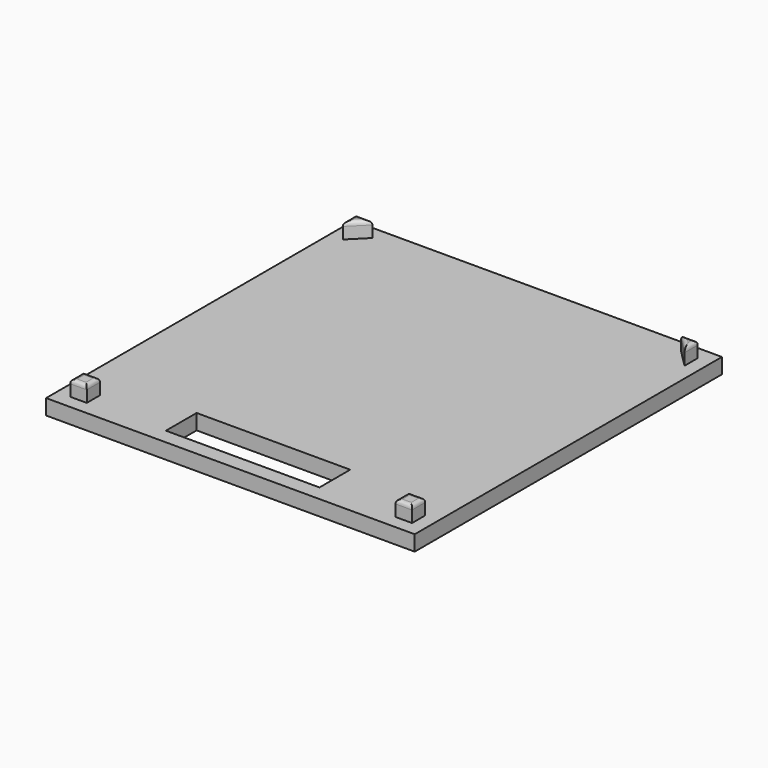
from build123d import *

# Parameters (mm, degrees)
F0_W         = 48
F0_H         = 50
F1_DEPTH     = 2
F3_DEPTH     = 2
F4_W         = 20
F4_H         = 5
F5_DEPTH     = 25
F6_T1_DEPTH  = 4.6464466094
F6_T3_DEPTH  = 4.6464466094
F6_T5_DEPTH  = 4.6464466094
F6_T7_DEPTH  = 5.5355339059
F6_T9_DEPTH  = 5.5355339059
F6_T11_DEPTH = 4.6464466094


# Not quite as in the source:
# - a fillet or chamfer that OpenCascade refuses, or shapes differently, is made with other operations: its cross-section is extruded or revolved along the edge and cut away or added
# - a feature names something its author has since deleted; it is built from what else it names


with BuildPart() as f1:
    # F0 (on Top) → F1 (new body)
    with BuildSketch(Plane.XY):
        with Locations((24, -25)):
            Rectangle(F0_W, F0_H)
    extrude(amount=F1_DEPTH)

    # F2 (on face) → F3 (join)
    with BuildSketch(Plane.XY.offset(2)):
        Polygon((1.75, -1.75), (1.75, -3.8964466094), (3.8964466094, -1.75), align=None)
        Polygon((44.1035533906, -1.75), (46.25, -3.8964466094), (46.25, -1.75), align=None)
        Polygon((46.25, -48.25), (46.25, -46.1035533906), (44.1035533906, -48.25), align=None)
        Polygon((3.8964466094, -48.25), (1.75, -46.1035533906), (1.75, -48.25), align=None)
        Polygon((3.8964466094, -46.1035533906), (1.75, -46.1035533906), (3.8964466094, -48.25), align=None)
        Polygon((44.1035533906, -48.25), (46.25, -46.1035533906), (44.1035533906, -46.1035533906), align=None)
    extrude(amount=F3_DEPTH)

    # F4 (on face) → F5 (cut)
    with BuildSketch(Plane.XY.offset(2)):
        with Locations((24, -45.5)):
            Rectangle(F4_W, F4_H)
    extrude(amount=-F5_DEPTH, mode=Mode.SUBTRACT)

    # F6: fillet of radius 0.5 on 14 edges, made by hand

    # F6_s2 → F6_t1 (cut)
    with BuildSketch(Plane.XZ.offset(44.8535533906)):
        with BuildLine():
            add(Edge.make_bspline(
                [(1.75, 3.5), (1.75, 4), (2.25, 4)],
                knots=[0, 0, 0, 1, 1, 1], degree=2, weights=[1, 1, 1]))
            Line((2.25, 4), (1.75, 4))
            Line((1.75, 4), (1.75, 3.5))
        make_face()
        with BuildLine():
            add(Edge.make_bspline(
                [(3.8964466094, 3.5), (3.8964466094, 4), (3.3964466094, 4)],
                knots=[0, 0, 0, 1, 1, 1], degree=2, weights=[1, 1, 1]))
            Line((3.3964466094, 4), (3.8964466094, 4))
            Line((3.8964466094, 4), (3.8964466094, 3.5))
        make_face()
        with BuildLine():
            add(Edge.make_bspline(
                [(46.25, 3.5), (46.25, 4), (45.75, 4)],
                knots=[0, 0, 0, 1, 1, 1], degree=2, weights=[1, 1, 1]))
            Line((45.75, 4), (46.25, 4))
            Line((46.25, 4), (46.25, 3.5))
        make_face()
        with BuildLine():
            add(Edge.make_bspline(
                [(44.1035533906, 3.5), (44.1035533906, 4), (44.6035533906, 4)],
                knots=[0, 0, 0, 1, 1, 1], degree=2, weights=[1, 1, 1]))
            Line((44.6035533906, 4), (44.1035533906, 4))
            Line((44.1035533906, 4), (44.1035533906, 3.5))
        make_face()
    extrude(amount=F6_T1_DEPTH, mode=Mode.SUBTRACT)

    # F6_s4 → F6_t3 (cut)
    with BuildSketch(Plane.YZ.offset(0.5)):
        with BuildLine():
            add(Edge.make_bspline(
                [(-48.25, 3.5), (-48.25, 4), (-47.75, 4)],
                knots=[0, 0, 0, 1, 1, 1], degree=2, weights=[1, 1, 1]))
            Line((-47.75, 4), (-48.25, 4))
            Line((-48.25, 4), (-48.25, 3.5))
        make_face()
        with BuildLine():
            add(Edge.make_bspline(
                [(-46.1035533906, 3.5), (-46.1035533906, 4), (-46.6035533906, 4)],
                knots=[0, 0, 0, 1, 1, 1], degree=2, weights=[1, 1, 1]))
            Line((-46.6035533906, 4), (-46.1035533906, 4))
            Line((-46.1035533906, 4), (-46.1035533906, 3.5))
        make_face()
        with BuildLine():
            add(Edge.make_bspline(
                [(-1.75, 3.5), (-1.75, 4), (-2.25, 4)],
                knots=[0, 0, 0, 1, 1, 1], degree=2, weights=[1, 1, 1]))
            Line((-2.25, 4), (-1.75, 4))
            Line((-1.75, 4), (-1.75, 3.5))
        make_face()
    extrude(amount=F6_T3_DEPTH, mode=Mode.SUBTRACT)

    # F6_s6 → F6_t5 (cut)
    with BuildSketch(Plane.XZ.offset(0.5)):
        with BuildLine():
            add(Edge.make_bspline(
                [(1.75, 3.5), (1.75, 4), (2.25, 4)],
                knots=[0, 0, 0, 1, 1, 1], degree=2, weights=[1, 1, 1]))
            Line((2.25, 4), (1.75, 4))
            Line((1.75, 4), (1.75, 3.5))
        make_face()
        with BuildLine():
            add(Edge.make_bspline(
                [(46.25, 3.5), (46.25, 4), (45.75, 4)],
                knots=[0, 0, 0, 1, 1, 1], degree=2, weights=[1, 1, 1]))
            Line((45.75, 4), (46.25, 4))
            Line((46.25, 4), (46.25, 3.5))
        make_face()
    extrude(amount=F6_T5_DEPTH, mode=Mode.SUBTRACT)

    # F6_s8 → F6_t7 (cut)
    with BuildSketch(Plane(origin=(-1.9571067812, -1.9571067812, 0), x_dir=(0, 0, 1), z_dir=(0.7071067812, 0.7071067812, 0))):
        with BuildLine():
            add(Edge.make_bspline(
                [(3.5, 3.9926406871), (4, 3.9926406871), (4, 3.4926406871)],
                knots=[0, 0, 0, 1, 1, 1], degree=2, weights=[1, 1, 1]))
            Line((4, 3.4926406871), (4, 3.9926406871))
            Line((4, 3.9926406871), (3.5, 3.9926406871))
        make_face()
    extrude(amount=F6_T7_DEPTH, mode=Mode.SUBTRACT)

    # F6_s10 → F6_t9 (cut)
    with BuildSketch(Plane(origin=(22.0428932188, -22.0428932188, 0), x_dir=(0, 0, 1), z_dir=(0.7071067812, -0.7071067812, 0))):
        with BuildLine():
            add(Edge.make_bspline(
                [(3.5, -29.9484848098), (4, -29.9484848098), (4, -30.4484848098)],
                knots=[0, 0, 0, 1, 1, 1], degree=2, weights=[1, 1, 1]))
            Line((4, -30.4484848098), (4, -29.9484848098))
            Line((4, -29.9484848098), (3.5, -29.9484848098))
        make_face()
    extrude(amount=F6_T9_DEPTH, mode=Mode.SUBTRACT)

    # F6_s12 → F6_t11 (cut)
    with BuildSketch(Plane.YZ.offset(42.8535533906)):
        with BuildLine():
            add(Edge.make_bspline(
                [(-1.75, 3.5), (-1.75, 4), (-2.25, 4)],
                knots=[0, 0, 0, 1, 1, 1], degree=2, weights=[1, 1, 1]))
            Line((-2.25, 4), (-1.75, 4))
            Line((-1.75, 4), (-1.75, 3.5))
        make_face()
        with BuildLine():
            add(Edge.make_bspline(
                [(-46.1035533906, 3.5), (-46.1035533906, 4), (-46.6035533906, 4)],
                knots=[0, 0, 0, 1, 1, 1], degree=2, weights=[1, 1, 1]))
            Line((-46.6035533906, 4), (-46.1035533906, 4))
            Line((-46.1035533906, 4), (-46.1035533906, 3.5))
        make_face()
        with BuildLine():
            add(Edge.make_bspline(
                [(-48.25, 3.5), (-48.25, 4), (-47.75, 4)],
                knots=[0, 0, 0, 1, 1, 1], degree=2, weights=[1, 1, 1]))
            Line((-47.75, 4), (-48.25, 4))
            Line((-48.25, 4), (-48.25, 3.5))
        make_face()
    extrude(amount=F6_T11_DEPTH, mode=Mode.SUBTRACT)


solid = f1.part
